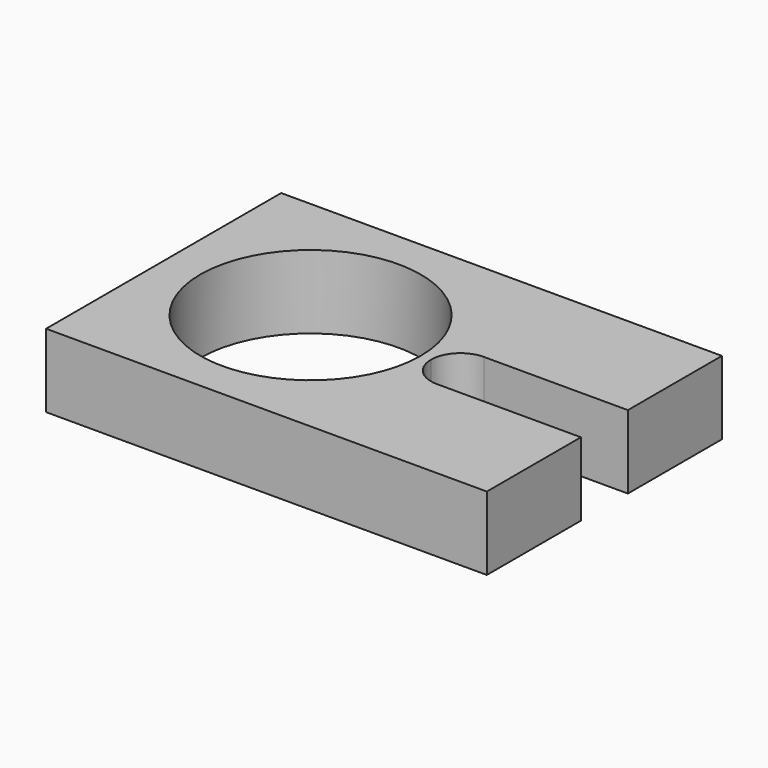
from build123d import *

# Parameters (mm, degrees)
F0_R     = 3.75
F1_DEPTH = 2.5
F2_R     = 1
F3_R     = 0.99999


# Not quite as in the source:
# - a fillet or chamfer is up to 0.001 mm smaller than in the source, because OpenCascade refuses the exact size


with BuildPart() as f1:
    # F0 (on Top) → F1 (new body)
    with BuildSketch(Plane.XY):
        Polygon((10, 5), (-5, 5), (-5, -5), (10, -5), (10, -2.5), (10, -1), (4.1, -1), (4.1, 1), (10, 1), (10, 2.5), align=None)
        Circle(F0_R, mode=Mode.SUBTRACT)
    extrude(amount=F1_DEPTH)

    # F2
    f2_edges = [f1.edges().sort_by_distance(p)[0] for p in [
        (4.1, 1, 1.25),
    ]]
    fillet(f2_edges, radius=F2_R)

    # F3 (radius 1 in the source; OpenCascade refuses exactly that, so slightly less here)
    f3_edges = [f1.edges().sort_by_distance(p)[0] for p in [
        (4.1, -1, 1.25),
    ]]
    fillet(f3_edges, radius=F3_R)


solid = f1.part
